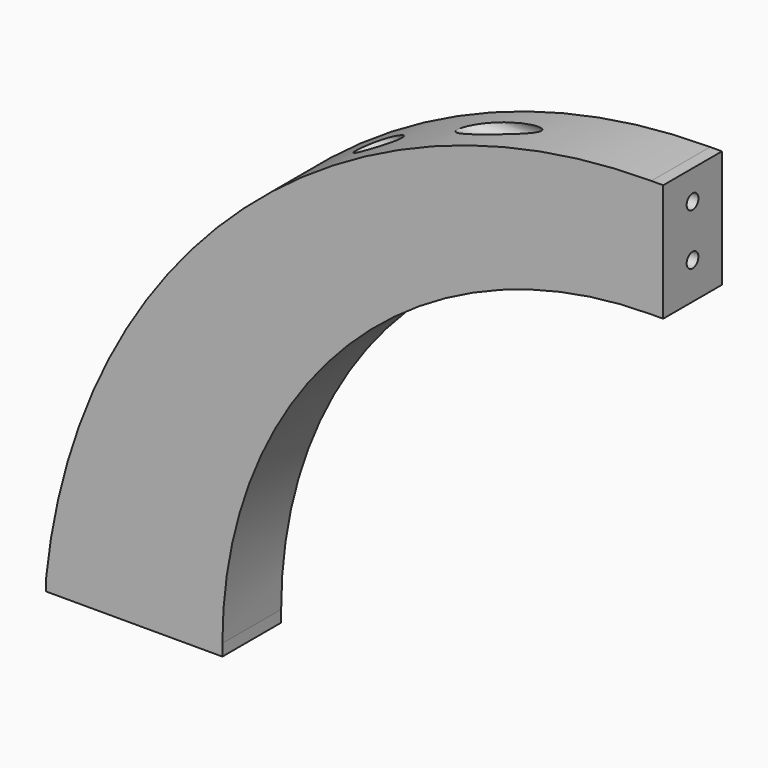
from build123d import *

# Parameters (mm, degrees)
F1_DEPTH      = 12.5
F2_R          = 2.5
F3_DEPTH      = 4
F4_R          = 4.5
F5_DEPTH      = 206.001
F6_R          = 3
F7_DEPTH      = 5
F8_R          = 6
F9_DEPTH      = 185.0010001
F10_S5_R      = 3
F10_T6_DEPTH  = 10
F10_S11_R     = 3
F10_T12_DEPTH = 10


# Not quite as in the source:
# - a fillet or chamfer that OpenCascade refuses, or shapes differently, is made with other operations: its cross-section is extruded or revolved along the edge and cut away or added


with BuildPart() as f1:
    # F0 (on Front) → F1 (new body, symmetric)
    with BuildSketch(Plane.XZ):
        with BuildLine():
            Line((0, 150), (0, 190))
            Line((0, 190), (-4, 190))
            ThreePointArc((-4, 190), (-142.7731962592, 136.6197765021), (-210, 4))
            Line((-210, 4), (-210, 0))
            Line((-210, 0), (-150, 0))
            Line((-150, 0), (-150, 4))
            ThreePointArc((-150, 4), (-107.2375900532, 107.2375900532), (-4, 150))
            Line((-4, 150), (0, 150))
        make_face()
    extrude(amount=F1_DEPTH, both=True)

    # F2 (on face) → F3 (cut)
    with BuildSketch(Plane.YZ):
        with Locations((0, 180)):
            Circle(F2_R)
        with Locations((0, 162.5)):
            Circle(F2_R)
    extrude(amount=-F3_DEPTH, mode=Mode.SUBTRACT)

    # F4 (on face) → F5 (cut, through all)
    with BuildSketch(Plane.YZ.offset(-4)):
        with Locations((0, 180)):
            Circle(F4_R)
        with Locations((0, 162.5)):
            Circle(F4_R)
    extrude(amount=-F5_DEPTH, mode=Mode.SUBTRACT)

    # F6 (on face) → F7 (cut)
    with BuildSketch(Plane(origin=(0, 0, 0), x_dir=(1, 0, 0), z_dir=(0, 0, -1))):
        with Locations((-165, 0)):
            Circle(F6_R)
        with Locations((-195, 0)):
            Circle(F6_R)
    extrude(amount=-F7_DEPTH, mode=Mode.SUBTRACT)

    # F8 (on face) → F9 (cut, through all)
    with BuildSketch(Plane(origin=(0, 0, 5), x_dir=(1, 0, 0), z_dir=(0, 0, -1))):
        with Locations((-165, 0)):
            Circle(F8_R)
        with Locations((-195, 0)):
            Circle(F8_R)
    extrude(amount=-F9_DEPTH, mode=Mode.SUBTRACT)

    # F10: chamfer of 5 on 2 edges, made by hand


with BuildPart() as f10_tool2:
    # F10_s3 → F10_t4 (revolve)
    with BuildSketch(Plane.XZ):
        Polygon((-189, 10), (-194, 5), (-189, 5), align=None)
    revolve(axis=Axis((-195, 0, 5), (0, 0, -1)))

    # F10_s5 → F10_t6 (cut, symmetric)
    with BuildSketch(Plane.XY.offset(7.5)):
        with Locations((-195, 0)):
            Circle(F10_S5_R)
    extrude(amount=F10_T6_DEPTH, both=True, mode=Mode.SUBTRACT)


with BuildPart() as f1_1:
    add(f1.part)

    # F10_t1: union F10_tool2
    add(f10_tool2.part)


with BuildPart() as f10_tool8:
    # F10_s9 → F10_t10 (revolve)
    with BuildSketch(Plane.XZ):
        Polygon((-159, 10), (-164, 5), (-159, 5), align=None)
    revolve(axis=Axis((-165, 0, 5), (0, 0, -1)))

    # F10_s11 → F10_t12 (cut, symmetric)
    with BuildSketch(Plane.XY.offset(7.5)):
        with Locations((-165, 0)):
            Circle(F10_S11_R)
    extrude(amount=F10_T12_DEPTH, both=True, mode=Mode.SUBTRACT)


with BuildPart() as f1_2:
    add(f1_1.part)

    # F10_t7: union F10_tool8
    add(f10_tool8.part)


solid = f1_2.part
